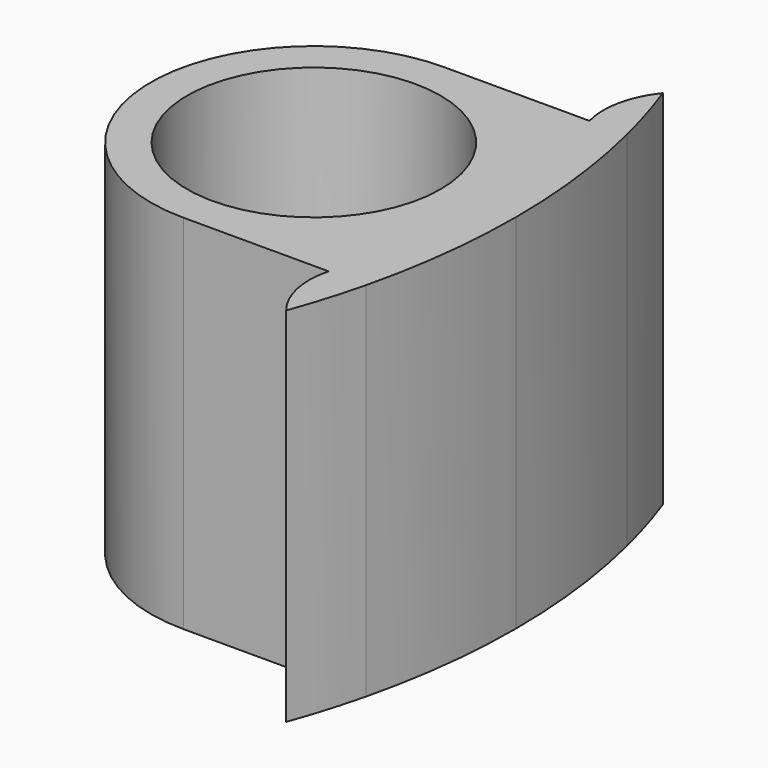
from build123d import *

# Parameters (mm, degrees)
F0_R        = 3.5
F1_DEPTH    = 10
F2_T1_DEPTH = 18.5839507528
F2_T3_DEPTH = 18.5839507528


# Not quite as in the source:
# - a fillet or chamfer that OpenCascade refuses, or shapes differently, is made with other operations: its cross-section is extruded or revolved along the edge and cut away or added


with BuildPart() as f1:
    # F0 (on Top) → F1 (new body)
    with BuildSketch(Plane.XY):
        with BuildLine():
            Line((17.4284250579, 4.5), (18.459414942, 4.5))
            ThreePointArc((18.459414942, 4.5), (18.1842599773, 5.507512059), (17.8541597949, 6.4983827232))
            Line((17.8541597949, 6.4983827232), (16.9144671741, 6.1563625799))
            ThreePointArc((16.9144671741, 6.1563625799), (17.191406166, 5.3343747558), (17.4284250579, 4.5))
        make_face()
        with BuildLine():
            ThreePointArc((17.8541597949, -6.4983827232), (18.1842599773, -5.507512059), (18.459414942, -4.5))
            Line((18.459414942, -4.5), (17.4284250579, -4.5))
            ThreePointArc((17.4284250579, -4.5), (17.191406166, -5.3343747558), (16.9144671741, -6.1563625799))
            Line((16.9144671741, -6.1563625799), (17.8541597949, -6.4983827232))
        make_face()
        with BuildLine():
            ThreePointArc((18.459414942, -4.5), (18.8643696409, -2.2661769682), (19, 0))
            ThreePointArc((19, 0), (18.8643696409, 2.2661769682), (18.459414942, 4.5))
            Line((18.459414942, 4.5), (17.4284250579, 4.5))
            ThreePointArc((17.4284250579, 4.5), (17.8565345328, 2.2680772647), (18, 0))
            ThreePointArc((18, 0), (17.8565345328, -2.2680772647), (17.4284250579, -4.5))
            Line((17.4284250579, -4.5), (18.459414942, -4.5))
        make_face()
        with BuildLine():
            ThreePointArc((18, 0), (17.8565345328, 2.2680772647), (17.4284250579, 4.5))
            Line((17.4284250579, 4.5), (13.4188298839, 4.5))
            ThreePointArc((13.4188298839, 4.5), (16.6008103993, 3.1819805153), (17.9188298839, 0))
            ThreePointArc((17.9188298839, 0), (16.6008103993, -3.1819805153), (13.4188298839, -4.5))
            Line((13.4188298839, -4.5), (17.4284250579, -4.5))
            ThreePointArc((17.4284250579, -4.5), (17.8565345328, -2.2680772647), (18, 0))
        make_face()
        with BuildLine():
            ThreePointArc((17.9188298839, 0), (16.6008103993, 3.1819805153), (13.4188298839, 4.5))
            ThreePointArc((13.4188298839, 4.5), (8.9188298839, 0), (13.4188298839, -4.5))
            ThreePointArc((13.4188298839, -4.5), (16.6008103993, -3.1819805153), (17.9188298839, 0))
        make_face()
        with Locations((13.4188298839, 0)):
            Circle(F0_R, mode=Mode.SUBTRACT)
    extrude(amount=F1_DEPTH)

    # F2: fillet of radius 2.25 on 2 edges, made by hand

    # F2_s2 → F2_t1 (cut)
    with BuildSketch(Plane.XY.offset(-4.2919753764)):
        with BuildLine():
            ThreePointArc((17.8541597949, 6.4983827232), (17.4032553622, 5.5588577913), (17.4240420287, 4.5169413745))
            ThreePointArc((17.4240420287, 4.5169413745), (17.1888111585, 5.342730665), (16.9144671741, 6.1563625799))
            Line((16.9144671741, 6.1563625799), (17.8541597949, 6.4983827232))
        make_face()
    extrude(amount=F2_T1_DEPTH, mode=Mode.SUBTRACT)

    # F2_s4 → F2_t3 (cut)
    with BuildSketch(Plane.XY.offset(-4.2919753764)):
        with BuildLine():
            ThreePointArc((17.8541597949, -6.4983827232), (17.4032553622, -5.5588577913), (17.4240420287, -4.5169413745))
            ThreePointArc((17.4240420287, -4.5169413745), (17.1888111585, -5.342730665), (16.9144671741, -6.1563625799))
            Line((16.9144671741, -6.1563625799), (17.8541597949, -6.4983827232))
        make_face()
    extrude(amount=F2_T3_DEPTH, mode=Mode.SUBTRACT)


solid = f1.part
